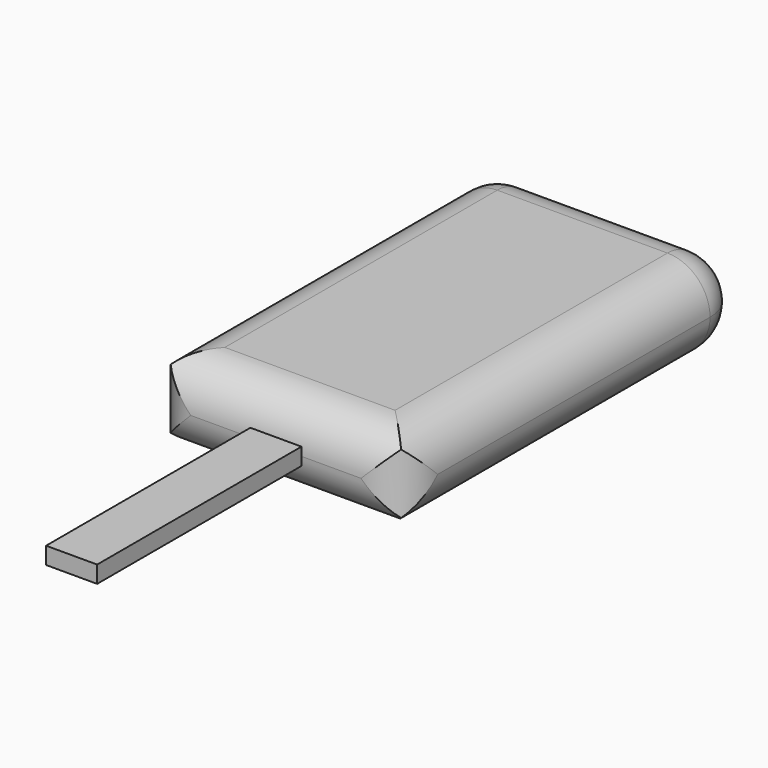
from build123d import *

# Parameters (mm, degrees)
F0_W        = 30
F0_H        = 50
F1_DEPTH    = 5
F2_R        = 4.99999
F3_W        = 6
F3_H        = 2
F4_DEPTH    = 30
F5_T1_DEPTH = 45.00002


# Not quite as in the source:
# - a fillet or chamfer that OpenCascade refuses, or shapes differently, is made with other operations: its cross-section is extruded or revolved along the edge and cut away or added
# - a fillet or chamfer is up to 0.001 mm smaller than in the source, because OpenCascade refuses the exact size


with BuildPart() as f1:
    # F0 (on Top) → F1 (new body, symmetric)
    with BuildSketch(Plane.XY):
        Rectangle(F0_W, F0_H)
    extrude(amount=F1_DEPTH, both=True)

    # F2 (radius 5 in the source; OpenCascade refuses exactly that, so slightly less here)
    f2_edges = [f1.edges().sort_by_distance(p)[0] for p in [
        (0, 25, -5),
        (-15, 25, 0),
        (0, 25, 5),
        (15, 25, 0),
        (-15, 0, -5),
        (-15, -25, 0),
        (-15, 0, 5),
        (15, 0, -5),
        (15, 0, 5),
        (15, -25, 0),
    ]]
    fillet(f2_edges, radius=F2_R)

    # F5: fillet of radius 5 on 8 edges, made by hand

    # F5_s2 → F5_t1 (cut)
    with BuildSketch(Plane.YZ.offset(-22.50001)):
        with BuildLine():
            ThreePointArc((-20, 5), (-23.5355339059, 3.5355339059), (-25, 0))
            Line((-25, 0), (-25, 5))
            Line((-25, 5), (-20, 5))
        make_face()
        with BuildLine():
            ThreePointArc((-20, -5), (-23.5355339059, -3.5355339059), (-25, 0))
            Line((-25, 0), (-25, -5))
            Line((-25, -5), (-20, -5))
        make_face()
    extrude(amount=F5_T1_DEPTH, mode=Mode.SUBTRACT)


with BuildPart() as f4:
    # F3 (on face) → F4 (new body)
    with BuildSketch(Plane.XZ.offset(25)):
        Rectangle(F3_W, F3_H)
    extrude(amount=F4_DEPTH)


solid = Compound([f1.part, f4.part])
